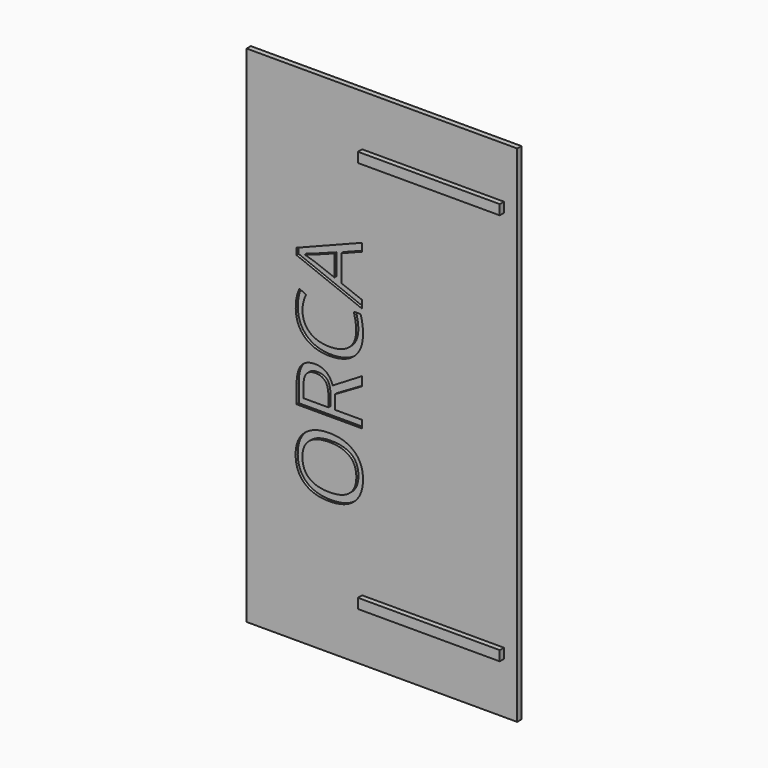
from build123d import *

# Parameters (mm, degrees)
F0_W         = 82
F0_H         = 153
F1_DEPTH     = 1.6
F3_W         = 43
F3_H         = 3
F4_DEPTH     = 1.6
F5_TEXT_SIZE = 27.7777777778
F6_DEPTH     = 0.8


# Not quite as in the source:
# - Text() gives the source's letters only with a copy of the font that has no kerning and outlines rounded to 1/6400 em; it was checked with that copy


with BuildPart() as f1:
    # F0 (on Front) → F1 (new body)
    with BuildSketch(Plane.XZ):
        with Locations((-41, 0)):
            Rectangle(F0_W, F0_H)
    extrude(amount=F1_DEPTH)

    # F3 (on offset) → F4 (join)
    with BuildSketch(Plane.XZ.offset(1.6)):
        with Locations((-25.5, 59.5)):
            Rectangle(F3_W, F3_H)
        with Locations((-25.5, -59.5)):
            Rectangle(F3_W, F3_H)
    extrude(amount=F4_DEPTH)

    # F5 (on face) → F6 (cut)
    with BuildSketch(Plane.XZ.offset(1.6)):
        with Locations(Location((-47, -37.8537326389), (0, 0, 90))):
            Text('ORCA', F5_TEXT_SIZE, font='Open Sans', text_align=(TextAlign.LEFT, TextAlign.BOTTOM))
    extrude(amount=-F6_DEPTH, mode=Mode.SUBTRACT)


solid = f1.part
